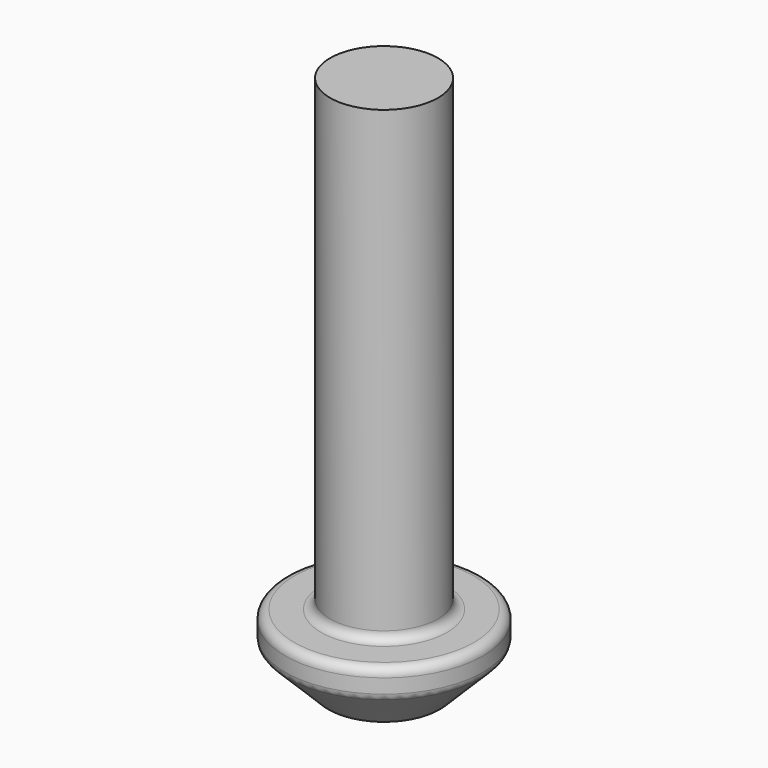
from build123d import *

# Parameters (mm, degrees)
F1_R     = 2.75
F1_R_2   = 1.5
F2_DEPTH = 2
F3_START = 1.5
F3_DEPTH = 0.5
F4_START = 2
F4_DEPTH = 13
F5_SIZE2 = 1.25
F5_SIZE  = 1.25
F6_R     = 0.25


# Not quite as in the source:
# - a feature names something its author has since deleted; it is built from what else it names


with BuildPart() as f2:
    # F1 (on Top) → F2 (new body)
    with BuildSketch(Plane.XY):
        Circle(F1_R)
        Circle(F1_R_2, mode=Mode.SUBTRACT)
        Circle(F1_R_2)
        Polygon((-0.5773502692, -1), (-1.1547005384, 0), (-0.5773502692, 1), (0.5773502692, 1), (1.1547005384, 0), (0.5773502692, -1), align=None, mode=Mode.SUBTRACT)
    extrude(amount=F2_DEPTH)

    # F1 (on Top) → F3 (join)
    with BuildSketch(Plane.XY.offset(F3_START)):
        Polygon((-0.5773502692, 1), (-1.1547005384, 0), (-0.5773502692, -1), (0.5773502692, -1), (1.1547005384, 0), (0.5773502692, 1), align=None)
    extrude(amount=F3_DEPTH)

    # F1 (on Top) → F4 (join)
    with BuildSketch(Plane.XY.offset(F4_START)):
        Circle(F1_R_2)
        Polygon((-0.5773502692, -1), (-1.1547005384, 0), (-0.5773502692, 1), (0.5773502692, 1), (1.1547005384, 0), (0.5773502692, -1), align=None, mode=Mode.SUBTRACT)
        Polygon((-0.5773502692, 1), (-1.1547005384, 0), (-0.5773502692, -1), (0.5773502692, -1), (1.1547005384, 0), (0.5773502692, 1), align=None)
    extrude(amount=F4_DEPTH)

    # F5
    f5_edges = [f2.edges().sort_by_distance(p)[0] for p in [
        (-2.75, 0, 0),
    ]]
    chamfer(f5_edges, length=F5_SIZE, length2=F5_SIZE2)

    # F6
    f6_edges = [f2.edges().sort_by_distance(p)[0] for p in [
        (-2.75, 0, 2),
        (-1.5, 0, 2),
        (-1.5, 0, 0),
        (-2.75, 0, 1.25),
    ]]
    fillet(f6_edges, radius=F6_R)


solid = f2.part
